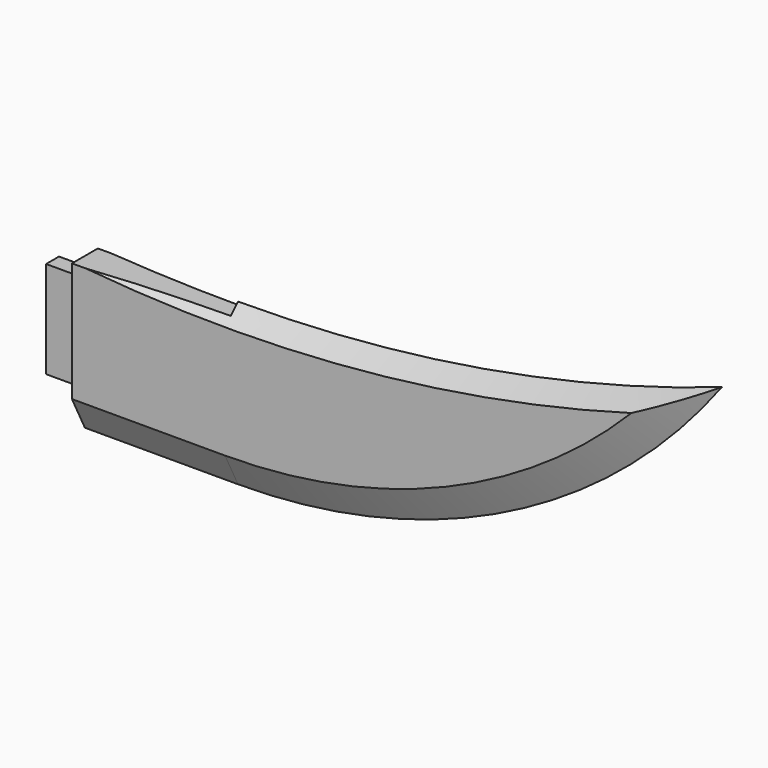
from build123d import *

# Parameters (mm, degrees)
F1_DEPTH    = 5
F2_DEPTH    = 5
F3_T2_ANGLE = 28.7632092252
F3_T4_ANGLE = 28.7632092252
F4_T1_DEPTH = 73.2511453801
F4_T4_ANGLE = 58.5309171072
F4_T6_ANGLE = 58.5309171072
F5_W        = 5
F5_H        = 30
F6_DEPTH    = 10


# Not quite as in the source:
# - a fillet or chamfer that OpenCascade refuses, or shapes differently, is made with other operations: its cross-section is extruded or revolved along the edge and cut away or added


with BuildPart() as f1:
    # F0 (on Front) → F1 (new body, symmetric)
    with BuildSketch(Plane.XZ):
        with BuildLine():
            Line((2.6443716172, -3.0652818078), (2.6443716172, -47.137426524))
            Line((2.6443716172, -47.137426524), (50, -47.137426524))
            ThreePointArc((50, -47.137426524), (128.4023811423, -29.5875675392), (191.8408584792, 19.7124376571))
            ThreePointArc((191.8408584792, 19.7124376571), (121.8130563717, 2.8164742266), (50, -2.862573476))
            Line((50, -2.862573476), (2.6443716172, -3.0652818078))
        make_face()
    extrude(amount=F1_DEPTH, both=True)

    # F0 (on Front) → F2 (join, symmetric)
    with BuildSketch(Plane.XZ):
        with BuildLine():
            Line((2.6443716172, -50), (50, -50))
            ThreePointArc((50, -50), (133.9633393999, -30.0622505081), (200, 25.494168336))
            ThreePointArc((200, 25.494168336), (127.7176805201, 6.7011176968), (53.3323914074, 0.0122294972))
            Line((53.3323914074, 0.0122294972), (50, -2.862573476))
            ThreePointArc((50, -2.862573476), (121.8130563717, 2.8164742266), (191.8408584792, 19.7124376571))
            ThreePointArc((191.8408584792, 19.7124376571), (128.4023811423, -29.5875675392), (50, -47.137426524))
            Line((50, -47.137426524), (2.6443716172, -47.137426524))
            Line((2.6443716172, -47.137426524), (2.6443716172, -50))
        make_face()
        Polygon((50, -2.862573476), (53.3323914074, 0.0122294972), (49.9881391504, -0.0917057033), align=None)
        with BuildLine():
            Line((2.6443716172, -3.0652818078), (2.6443716172, -47.137426524))
            Line((2.6443716172, -47.137426524), (50, -47.137426524))
            ThreePointArc((50, -47.137426524), (128.4023811423, -29.5875675392), (191.8408584792, 19.7124376571))
            ThreePointArc((191.8408584792, 19.7124376571), (121.8130563717, 2.8164742266), (50, -2.862573476))
            Line((50, -2.862573476), (2.6443716172, -3.0652818078))
        make_face()
    extrude(amount=F2_DEPTH, both=True)

    # F3: chamfer of 5.08 on 2 edges, made by hand

    # F3_s1 → F3_t2 (revolve, cut)
    with BuildSketch(Plane(origin=(195.1630456204, 0, 74.6833379712), x_dir=(0, 1, 0), z_dir=(0.9339525469, 0, 0.3573970343))):
        Polygon((-5, -52.9370117112), (0.08, -47.8570117112), (-5, -47.8570117112), align=None)
    revolve(axis=Axis((50, -5, 454.0244716756), (0, 1, 0)), revolution_arc=F3_T2_ANGLE, mode=Mode.SUBTRACT)

    # F3_s3 → F3_t4 (revolve, cut)
    with BuildSketch(Plane(origin=(195.1630456204, 0, 74.6833379712), x_dir=(0, 1, 0), z_dir=(0.9339525469, 0, 0.3573970343))):
        Polygon((-0.08, -47.8570117112), (5, -52.9370117112), (5, -47.8570117112), align=None)
    revolve(axis=Axis((50, 5, 454.0244716756), (0, 1, 0)), revolution_arc=F3_T4_ANGLE, mode=Mode.SUBTRACT)

    # F4: chamfer of 5.08 x 10 on 2 edges, made by hand

    # F4_s2 → F4_t1 (cut)
    with BuildSketch(Plane.YZ.offset(-23.2511453801)):
        Polygon((0.08, -50), (-5, -40), (-5, -50), align=None)
        Polygon((5, -40), (-0.08, -50), (5, -50), align=None)
    extrude(amount=F4_T1_DEPTH, mode=Mode.SUBTRACT)

    # F4_s3 → F4_t4 (revolve, cut)
    with BuildSketch(Plane.YZ.offset(50)):
        Polygon((5, -40), (-0.08, -50), (5, -50), align=None)
    revolve(axis=Axis((50, 5, 136.7652169319), (0, -1, 0)), revolution_arc=F4_T4_ANGLE, mode=Mode.SUBTRACT)

    # F4_s5 → F4_t6 (revolve, cut)
    with BuildSketch(Plane.YZ.offset(50)):
        Polygon((-5, -40), (0.08, -50), (-5, -50), align=None)
    revolve(axis=Axis((50, -5, 136.7652169319), (0, -1, 0)), revolution_arc=F4_T6_ANGLE, mode=Mode.SUBTRACT)

    # F5 (on face) → F6 (join)
    with BuildSketch(Plane(origin=(2.6443716172, 0, 0), x_dir=(0, -1, 0), z_dir=(-1, 0, 0))):
        with Locations((0, -22.5)):
            Rectangle(F5_W, F5_H)
    extrude(amount=F6_DEPTH)


solid = f1.part
